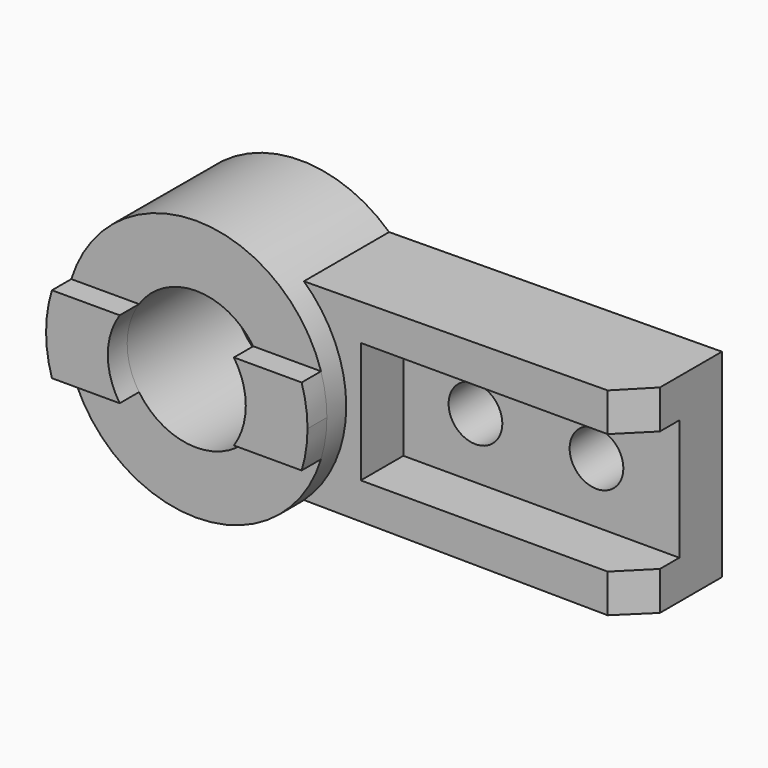
from build123d import *

# Parameters (mm, degrees)
F0_R      = 54
F0_R_2    = 28.5
F1_DEPTH  = 54
F3_DEPTH  = 10
F5_DEPTH  = 44
F6_W      = 114
F6_H      = 50
F7_DEPTH  = 22
F8_SIZE   = 12
F9_R      = 11.1
F10_DEPTH = 22


# Not quite as in the source:
# - after a boolean that leaves OpenCascade's solid faulty, fix() repairs it


with BuildPart() as f1:
    # F0 (on Front) → F1 (new body)
    with BuildSketch(Plane.XZ):
        Circle(F0_R)
        Circle(F0_R_2, mode=Mode.SUBTRACT)
    extrude(amount=F1_DEPTH)

    # F2 (on face) → F3 (join)
    with BuildSketch(Plane.XZ.offset(54)):
        with BuildLine():
            Line((-23.5849528301, 16), (-51.5751878329, 16))
            ThreePointArc((-51.5751878329, 16), (-54, 0), (-51.5751878329, -16))
            Line((-51.5751878329, -16), (-23.5849528301, -16))
            ThreePointArc((-23.5849528301, -16), (-28.5, 0), (-23.5849528301, 16))
        make_face()
        with BuildLine():
            ThreePointArc((51.5751878329, -16), (53.3903556037, -8.0913489921), (54, 0))
            ThreePointArc((54, 0), (53.3903556037, 8.0913489921), (51.5751878329, 16))
            Line((51.5751878329, 16), (23.5849528301, 16))
            ThreePointArc((23.5849528301, 16), (27.2435419472, 8.368955859), (28.5, 0))
            ThreePointArc((28.5, 0), (27.2435419472, -8.368955859), (23.5849528301, -16))
            Line((23.5849528301, -16), (51.5751878329, -16))
        make_face()
    extrude(amount=F3_DEPTH)

    add(f1.part.fix(), mode=Mode.REPLACE)

    # F4 (on face) → F5 (join)
    with BuildSketch(Plane(origin=(0, 0, 0), x_dir=(-1, 0, 0), z_dir=(0, 1, 0))):
        with BuildLine():
            Line((-174, 41), (-174, 0))
            Line((-174, 0), (-174, -41))
            Line((-174, -41), (-36.5173199288, -39.7804643666))
            ThreePointArc((-36.5173199288, -39.7804643666), (-54, 0), (-36.5173199288, 39.7804643666))
            Line((-36.5173199288, 39.7804643666), (-174, 41))
        make_face()
    extrude(amount=-F5_DEPTH)

    # F6 (on face) → F7 (cut)
    with BuildSketch(Plane.XZ.offset(44)):
        with Locations((117, 0)):
            Rectangle(F6_W, F6_H)
    extrude(amount=-F7_DEPTH, mode=Mode.SUBTRACT)

    # F8
    f8_edges = [f1.edges().sort_by_distance(p)[0] for p in [
        (174, -44, 33),
        (174, -44, -33),
    ]]
    chamfer(f8_edges, length=F8_SIZE)

    # F9 (on face) → F10 (cut, through all)
    with BuildSketch(Plane.XZ.offset(22)):
        with Locations((139.781537652, 0)):
            Circle(F9_R)
        with Locations((89.781537652, 0)):
            Circle(F9_R)
    extrude(amount=-F10_DEPTH, mode=Mode.SUBTRACT)


solid = f1.part
